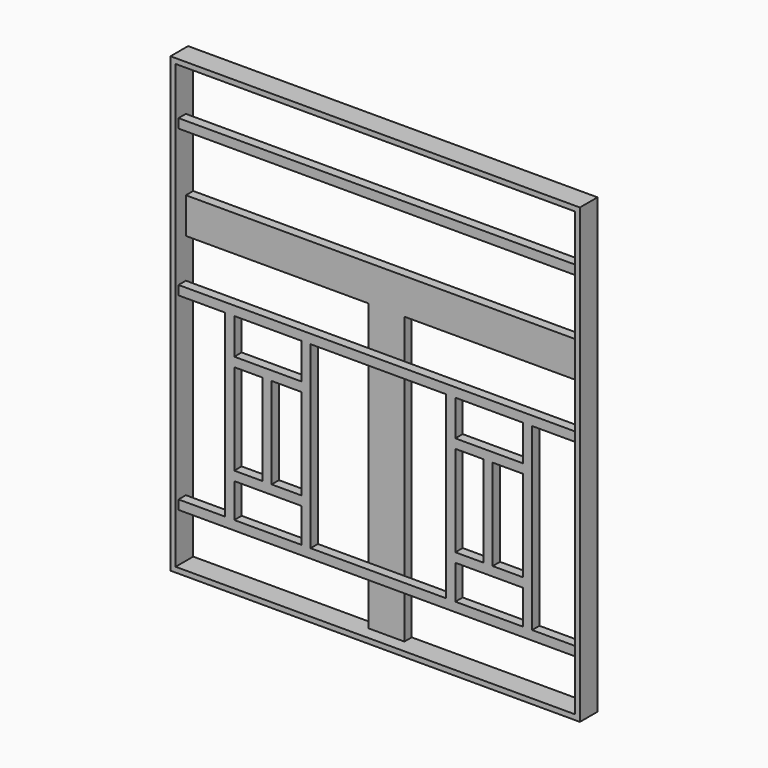
from build123d import *

# Parameters (mm, degrees)
F0_W     = 55
F0_H     = 178
F0_W_2   = 58
F0_W_3   = 59
F0_W_4   = 70
F0_H_2   = 18
F1_DEPTH = 18
F0_W_5   = 780
F0_W_6   = 800
F0_H_3   = 885
F2_DEPTH = 25
F0_W_7   = 357
F0_H_4   = 70
F0_W_8   = 353
F0_H_5   = 351
F0_H_6   = 95
F0_H_7   = 77
F3_DEPTH = 18


# Not quite as in the source:
# - a feature names something its author has since deleted; it is built from what else it names


with BuildPart() as f1:
    # F0 (on Front) → F1 (new body)
    with BuildSketch(Plane.XZ):
        Polygon((-299, 49.5), (-390, 49.5), (-390, 40.5200137198), (-390, 31.5), (-299, 31.5), (-299, -38.5), (-299, -56.5), (-299, -234.5), (-299, -252.5), (-299, -319.5), (-390, -319.5), (-390, -337.5), (-299, -337.5), (-281, -337.5), (-150, -337.5), (-132, -337.5), (-33, -337.5), (-33, -319.5), (-132, -319.5), (-132, -252.5), (-132, -234.5), (-132, -56.5), (-132, -38.5), (-132, 31.5), (-33, 31.5), (-33, 49.5), (-132, 49.5), (-150, 49.5), (-281, 49.5), align=None)
        Polygon((-226, -252.5), (-208, -252.5), (-150, -252.5), (-150, -319.5), (-281, -319.5), (-281, -252.5), align=None, mode=Mode.SUBTRACT)
        with Locations((-253.5, -145.5)):
            Rectangle(F0_W, F0_H, mode=Mode.SUBTRACT)
        Polygon((-281, 31.5), (-150, 31.5), (-150, -38.5), (-208, -38.5), (-226, -38.5), (-281, -38.5), align=None, mode=Mode.SUBTRACT)
        with Locations((-179, -145.5)):
            Rectangle(F0_W_2, F0_H, mode=Mode.SUBTRACT)
        Polygon((390, 40.5200137198), (390, 49.5), (301, 49.5), (283, 49.5), (151, 49.5), (133, 49.5), (37, 49.5), (37, 31.5), (133, 31.5), (133, -38.5), (133, -56.5), (133, -234.5), (133, -252.5), (133, -319.5), (37, -319.5), (37, -337.5), (133, -337.5), (151, -337.5), (283, -337.5), (301, -337.5), (390, -337.5), (390, -319.5), (301, -319.5), (301, -252.5), (301, -234.5), (301, -56.5), (301, -38.5), (301, 31.5), (390, 31.5), align=None)
        Polygon((206, -252.5), (224, -252.5), (283, -252.5), (283, -319.5), (151, -319.5), (151, -252.5), align=None, mode=Mode.SUBTRACT)
        with Locations((178.5, -145.5)):
            Rectangle(F0_W, F0_H, mode=Mode.SUBTRACT)
        with Locations((253.5, -145.5)):
            Rectangle(F0_W_3, F0_H, mode=Mode.SUBTRACT)
        Polygon((151, 31.5), (283, 31.5), (283, -38.5), (224, -38.5), (206, -38.5), (151, -38.5), align=None, mode=Mode.SUBTRACT)
        with Locations((2, 40.5)):
            Rectangle(F0_W_4, F0_H_2)
        with Locations((2, -328.5)):
            Rectangle(F0_W_4, F0_H_2)
    extrude(amount=F1_DEPTH)



with BuildPart() as f1b:
    # F0 (on Front) → F1, piece 2 (new body)
    with BuildSketch(Plane.XZ):
        with Locations((0, 327.5)):
            Rectangle(F0_W_5, F0_H_2)
    extrude(amount=F1_DEPTH)


with BuildPart() as f1_1:
    add(f1.part)

    add(f1b.part)  # F2 merges F1b
    # F0 (on Front) → F2 (join)
    with BuildSketch(Plane.XZ):
        Rectangle(F0_W_6, F0_H_3)
        Polygon((-390, 432.5), (390, 432.5), (390, 336.5), (390, 318.5), (390, 196.5), (390, 126.5), (390, 49.5), (390, 40.5200137198), (390, 31.5), (390, -38.5), (390, -56.5), (390, -234.5), (390, -252.5), (390, -319.5), (390, -337.5), (390, -432.5), (37, -432.5), (-33, -432.5), (-390, -432.5), (-390, -337.5), (-390, -319.5), (-390, -252.5), (-390, -234.5), (-390, -140.5), (-390, -56.5), (-390, -38.5), (-390, 31.5), (-390, 40.5200137198), (-390, 49.5), (-390, 126.5), (-390, 196.5), (-390, 318.5), (-390, 336.5), align=None, mode=Mode.SUBTRACT)
    extrude(amount=F2_DEPTH)

    # F0 (on Front) → F3 (join)
    with BuildSketch(Plane.XZ):
        Rectangle(F0_W_6, F0_H_3)
        Polygon((-390, 432.5), (390, 432.5), (390, 336.5), (390, 318.5), (390, 196.5), (390, 126.5), (390, 49.5), (390, 40.5200137198), (390, 31.5), (390, -38.5), (390, -56.5), (390, -234.5), (390, -252.5), (390, -319.5), (390, -337.5), (390, -432.5), (37, -432.5), (-33, -432.5), (-390, -432.5), (-390, -337.5), (-390, -319.5), (-390, -252.5), (-390, -234.5), (-390, -140.5), (-390, -56.5), (-390, -38.5), (-390, 31.5), (-390, 40.5200137198), (-390, 49.5), (-390, 126.5), (-390, 196.5), (-390, 318.5), (-390, 336.5), align=None, mode=Mode.SUBTRACT)
        with Locations((-211.5, 161.5)):
            Rectangle(F0_W_7, F0_H_4)
        with Locations((213.5, 161.5)):
            Rectangle(F0_W_8, F0_H_4)
        with Locations((2, -144)):
            Rectangle(F0_W_4, F0_H_5)
        with Locations((2, -385)):
            Rectangle(F0_W_4, F0_H_6)
        with Locations((2, 88)):
            Rectangle(F0_W_4, F0_H_7)
        with Locations((2, 161.5)):
            Rectangle(F0_W_4, F0_H_4)
        with Locations((2, 40.5)):
            Rectangle(F0_W_4, F0_H_2)
        with Locations((2, -328.5)):
            Rectangle(F0_W_4, F0_H_2)
    extrude(amount=-F3_DEPTH)


solid = f1_1.part
